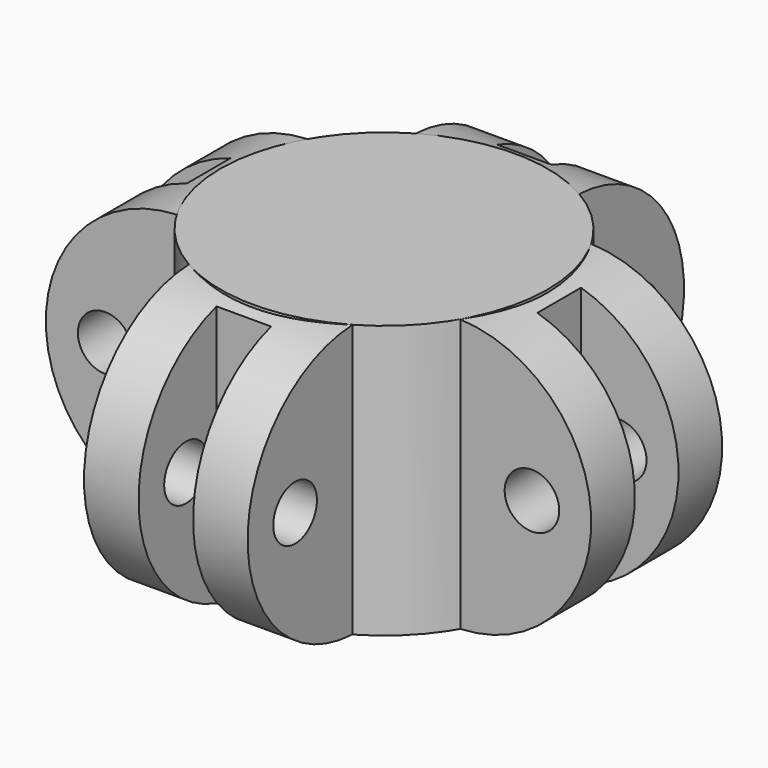
from build123d import *

# Parameters (mm, degrees)
F0_W            = 25
F0_H            = 50
F0_R            = 5
F1_DEPTH        = 15
F1_DEPTH_BACK   = 15
F2_COUNT        = 2
F2_ANGLE        = 90
F3_R            = 30
F4_DEPTH        = 50
F5_W            = 10
F5_H            = 64.0000030398
F6_DEPTH        = 50.0010001
F6_COPIES_COUNT = 4


# Not quite as in the source:
# - a pattern or mirror of a feature is missing from the dataset's text; its kind, count and spacing are read off the source's solid


with BuildPart() as f1:
    # F0 (on Front) → F1 (new body, two sides)
    with BuildSketch(Plane.XZ) as f1_sk:
        with Locations((-12.5, 25)):
            Rectangle(F0_W, F0_H)
        with Locations((12.5, 25)):
            Rectangle(F0_W, F0_H)
        with BuildLine():
            ThreePointArc((-25, 50), (-50, 25), (-25, 0))
            Line((-25, 0), (-25, 50))
        make_face()
        with Locations((-39.1249991953, 25)):
            Circle(F0_R, mode=Mode.SUBTRACT)
        with BuildLine():
            Line((25, 50), (25, 0))
            ThreePointArc((25, 0), (50, 25), (25, 50))
        make_face()
        with Locations((39.1249991953, 25)):
            Circle(F0_R, mode=Mode.SUBTRACT)
    extrude(amount=F1_DEPTH)
    extrude(f1_sk.sketch, amount=-F1_DEPTH_BACK)

    # F2: F1 ×2 about axis
    f2_axis = Axis((0, 0, 10.6249991804), (0, 0, 1))


with BuildPart() as f1_1:
    add(f1.part)
    for i in range(1, F2_COUNT):
        add(f1.part.rotate(f2_axis, i * F2_ANGLE / (F2_COUNT - 1)))

    # F3 (on face) → F4 (join, through all)
    with BuildSketch(Plane.XY.offset(50)):
        Circle(F3_R)
    extrude(amount=-F4_DEPTH)

    # F5 (on face) → F6 (cut, through all)
    with BuildSketch(Plane.XY.offset(50)):
        with Locations((0, 64.1250014305)):
            Rectangle(F5_W, F5_H)
    f6 = extrude(amount=-F6_DEPTH, mode=Mode.SUBTRACT)

    # F6_copies: F6 ×4 about axis
    f6_copies_axis = Axis((0, 0, 0), (0, 0, 1))
    for i in range(1, F6_COPIES_COUNT):
        add(f6.rotate(f6_copies_axis, i * 360 / F6_COPIES_COUNT), mode=Mode.SUBTRACT)


solid = f1_1.part
